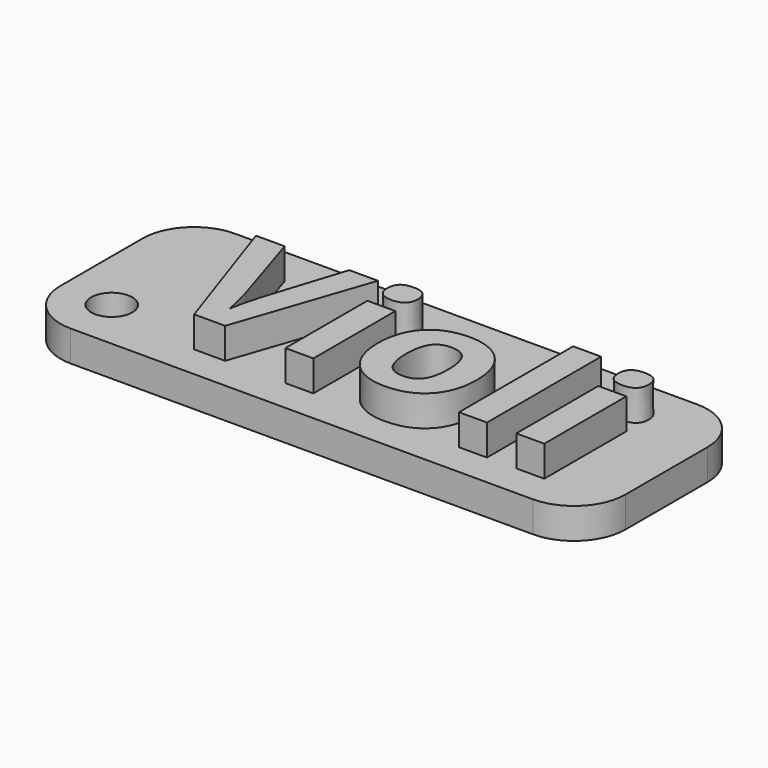
from build123d import *

# Parameters (mm, degrees)
F0_W         = 55
F0_H         = 20
F1_DEPTH     = 3
F2_TEXT_SIZE = 18.2823892424
F3_DEPTH     = 3
F4_R         = 5
F5_R         = 2
F6_DEPTH     = 25


# Not quite as in the source:
# - Text() gives the source's letters only with a copy of the font that has no kerning and outlines rounded to 1/6400 em; it was checked with that copy


with BuildPart() as f1:
    # F0 (on Top) → F1 (new body)
    with BuildSketch(Plane.XY):
        with Locations((-15.7274080813, -2.8896264359)):
            Rectangle(F0_W, F0_H)
    extrude(amount=F1_DEPTH)

    # F2 (on face) → F3 (join)
    with BuildSketch(Plane.XY.offset(3)):
        with Locations((-33.1829104107, -9.7050721524)):
            Text('Violi', F2_TEXT_SIZE, font='Open Sans', font_style=FontStyle.BOLD, text_align=(TextAlign.LEFT, TextAlign.BOTTOM))
    extrude(amount=F3_DEPTH)

    # F4
    f4_edges = [f1.edges().sort_by_distance(p)[0] for p in [
        (-43.227408, 7.110374, 1.5),
        (-43.227408, -12.889626, 1.5),
        (11.772592, -12.889626, 1.5),
        (11.772592, 7.110374, 1.5),
    ]]
    fillet(f4_edges, radius=F4_R)

    # F5 (on face) → F6 (cut)
    with BuildSketch(Plane.XY.offset(3)):
        with Locations((-38.2274080813, -7.8896264359)):
            Circle(F5_R)
    extrude(amount=-F6_DEPTH, mode=Mode.SUBTRACT)


solid = f1.part
